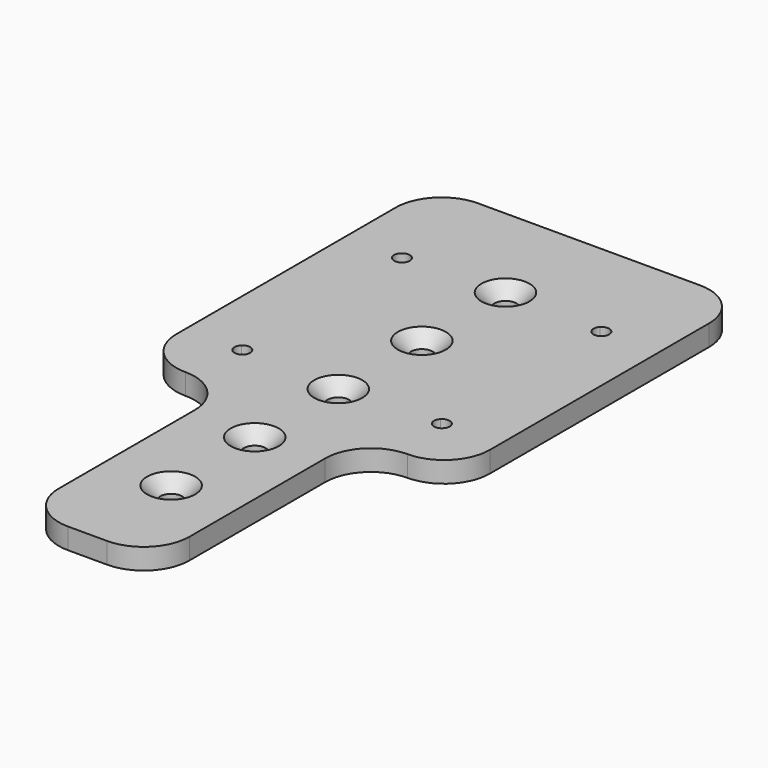
from build123d import *

# Parameters (mm, degrees)
F0_W     = 60
F0_H     = 160
F1_DEPTH = 4
F2_W     = 60
F2_H     = 40
F3_DEPTH = 4.001
F4_R     = 2.1
F5_DEPTH = 4.001
F6_SIZE  = 2.5
F7_W     = 17.5
F7_H     = 50
F8_DEPTH = 4.001
F9_R     = 8.74999


# Not quite as in the source:
# - a fillet or chamfer is up to 0.001 mm smaller than in the source, because OpenCascade refuses the exact size


with BuildPart() as f1:
    # F0 (on Top) → F1 (new body)
    with BuildSketch(Plane.XY):
        Rectangle(F0_W, F0_H)
        with BuildLine():
            ThreePointArc((20.122671197, 18.002169422), (25.2221343498, 9.6355559695), (27, 0))
            ThreePointArc((27, 0), (25.2221343498, -9.6355559695), (20.122671197, -18.002169422))
            ThreePointArc((20.122671197, -18.002169422), (20.4695953547, -18.4986639746), (20.591883092, -19.091883092))
            ThreePointArc((20.591883092, -19.091883092), (19.6466035148, -20.4855420362), (18.002169422, -20.122671197))
            ThreePointArc((18.002169422, -20.122671197), (0, -27), (-18.002169422, -20.122671197))
            ThreePointArc((-18.002169422, -20.122671197), (-20.1525432638, -20.1525432638), (-20.122671197, -18.002169422))
            ThreePointArc((-20.122671197, -18.002169422), (-27, 0), (-20.122671197, 18.002169422))
            ThreePointArc((-20.122671197, 18.002169422), (-20.1525432638, 20.1525432638), (-18.002169422, 20.122671197))
            ThreePointArc((-18.002169422, 20.122671197), (0, 27), (18.002169422, 20.122671197))
            ThreePointArc((18.002169422, 20.122671197), (19.6466035148, 20.4855420362), (20.591883092, 19.091883092))
            ThreePointArc((20.591883092, 19.091883092), (20.4695953547, 18.4986639746), (20.122671197, 18.002169422))
        make_face(mode=Mode.SUBTRACT)
        with BuildLine():
            Line((-18.0312229203, -18.0312229203), (0, 0))
            Line((0, 0), (-18.0312229203, 18.0312229203))
            ThreePointArc((-18.0312229203, 18.0312229203), (-19.0710477486, 17.5920278029), (-20.122671197, 18.002169422))
            ThreePointArc((-20.122671197, 18.002169422), (-27, 0), (-20.122671197, -18.002169422))
            ThreePointArc((-20.122671197, -18.002169422), (-19.0710477486, -17.5920278029), (-18.0312229203, -18.0312229203))
        make_face()
        with BuildLine():
            Line((0, 0), (18.0312229203, 18.0312229203))
            ThreePointArc((18.0312229203, 18.0312229203), (17.5920278029, 19.0710477486), (18.002169422, 20.122671197))
            ThreePointArc((18.002169422, 20.122671197), (0, 27), (-18.002169422, 20.122671197))
            ThreePointArc((-18.002169422, 20.122671197), (-17.6982241479, 19.6466035148), (-17.591883092, 19.091883092))
            ThreePointArc((-17.591883092, 19.091883092), (-17.7060637933, 18.5178579435), (-18.0312229203, 18.0312229203))
            Line((-18.0312229203, 18.0312229203), (0, 0))
        make_face()
        with BuildLine():
            ThreePointArc((20.122671197, -18.002169422), (25.2221343498, -9.6355559695), (27, 0))
            ThreePointArc((27, 0), (25.2221343498, 9.6355559695), (20.122671197, 18.002169422))
            ThreePointArc((20.122671197, 18.002169422), (19.0710477486, 17.5920278029), (18.0312229203, 18.0312229203))
            Line((18.0312229203, 18.0312229203), (0, 0))
            Line((0, 0), (18.0312229203, -18.0312229203))
            ThreePointArc((18.0312229203, -18.0312229203), (19.0710477486, -17.5920278029), (20.122671197, -18.002169422))
        make_face()
        with BuildLine():
            ThreePointArc((18.002169422, -20.122671197), (17.5920278029, -19.0710477486), (18.0312229203, -18.0312229203))
            Line((18.0312229203, -18.0312229203), (0, 0))
            Line((0, 0), (-18.0312229203, -18.0312229203))
            ThreePointArc((-18.0312229203, -18.0312229203), (-17.7060637933, -18.5178579435), (-17.591883092, -19.091883092))
            ThreePointArc((-17.591883092, -19.091883092), (-17.6982241479, -19.6466035148), (-18.002169422, -20.122671197))
            ThreePointArc((-18.002169422, -20.122671197), (0, -27), (18.002169422, -20.122671197))
        make_face()
    extrude(amount=F1_DEPTH)

    # F2 (on face) → F3 (cut, through all)
    with BuildSketch(Plane.XY.offset(4)):
        with Locations((0, 60)):
            Rectangle(F2_W, F2_H)
    extrude(amount=-F3_DEPTH, mode=Mode.SUBTRACT)

    # F4 (on face) → F5 (cut, through all)
    with BuildSketch(Plane(origin=(0, 0, 0), x_dir=(1, 0, 0), z_dir=(0, 0, -1))):
        with Locations((0, 40)):
            Circle(F4_R)
        Circle(F4_R)
        with Locations((0, 20)):
            Circle(F4_R)
        with Locations((0, -20)):
            Circle(F4_R)
        with Locations((0, 60)):
            Circle(F4_R)
    extrude(amount=-F5_DEPTH, mode=Mode.SUBTRACT)

    # F6
    f6_edges = [f1.edges().sort_by_distance(p)[0] for p in [
        (-2.1, -60, 4),
        (-2.1, -40, 4),
        (-2.1, -20, 4),
        (-2.1, 0, 4),
        (-2.1, 20, 4),
    ]]
    chamfer(f6_edges, length=F6_SIZE)

    # F7 (on face) → F8 (cut, through all)
    with BuildSketch(Plane(origin=(0, 0, 0), x_dir=(1, 0, 0), z_dir=(0, 0, -1))):
        with Locations((-21.25, 55)):
            Rectangle(F7_W, F7_H)
        with Locations((21.25, 55)):
            Rectangle(F7_W, F7_H)
    extrude(amount=-F8_DEPTH, mode=Mode.SUBTRACT)

    # F9 (radius 8.75 in the source; OpenCascade refuses exactly that, so slightly less here)
    f9_edges = [f1.edges().sort_by_distance(p)[0] for p in [
        (-12.5, -30, 2),
        (-30, -30, 2),
        (12.5, -30, 2),
        (30, -30, 2),
        (-30, 40, 2),
        (30, 40, 2),
        (-12.5, -80, 2),
        (12.5, -80, 2),
    ]]
    fillet(f9_edges, radius=F9_R)


solid = f1.part
